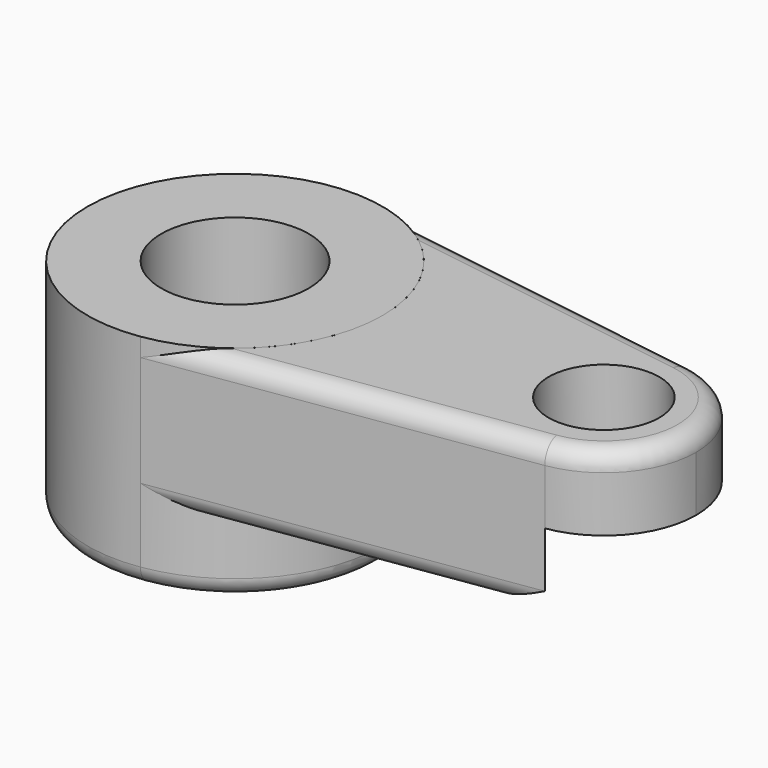
from build123d import *

# Parameters (mm, degrees)
F0_R         = 20
F1_DEPTH     = 60
F2_DEPTH     = 40
F0_R_2       = 15
F3_DEPTH     = 20
F4_R         = 5
F5_T1_DEPTH  = 141.3685996664
F5_T3_DEPTH  = 141.3685996664
F5_T5_DEPTH  = 120.1185996664
F5_T7_DEPTH  = 120.1185996664
F5_T10_ANGLE = 162.7461468826


# Not quite as in the source:
# - a fillet or chamfer that OpenCascade refuses, or shapes differently, is made with other operations: its cross-section is extruded or revolved along the edge and cut away or added
# - two fillets or chamfers of one size are made in one step


with BuildPart() as f1:
    # F0 (on Top) → F1 (new body)
    with BuildSketch(Plane.XY):
        with BuildLine():
            ThreePointArc((-44, -39.5474398666), (-19.6684982238, -26.0768096208), (-10, 0))
            ThreePointArc((-10, 0), (-19.6684982238, 26.0768096208), (-44, 39.5474398666))
            ThreePointArc((-44, 39.5474398666), (-90, 0), (-44, -39.5474398666))
        make_face()
        with Locations((-50, 0)):
            Circle(F0_R, mode=Mode.SUBTRACT)
    extrude(amount=-F1_DEPTH)

    # F4
    f4_edges = [f1.edges().sort_by_distance(p)[0] for p in [
        (-56, 39.54744, -60),
        (-70, 0, -60),
    ]]
    fillet(f4_edges, radius=F4_R)


with BuildPart() as f2:
    # F0 (on Top) → F2 (new body)
    with BuildSketch(Plane.XY):
        with BuildLine():
            ThreePointArc((-44, 39.5474398666), (-19.6684982238, 26.0768096208), (-10, 0))
            ThreePointArc((-10, 0), (-19.6684982238, -26.0768096208), (-44, -39.5474398666))
            Line((-44, -39.5474398666), (53.75, -24.7171499166))
            ThreePointArc((53.75, -24.7171499166), (25, 0), (53.75, 24.7171499166))
            Line((53.75, 24.7171499166), (-44, 39.5474398666))
        make_face()
    extrude(amount=-F2_DEPTH)

    # F0 (on Top) → F3 (join)
    with BuildSketch(Plane.XY):
        with BuildLine():
            ThreePointArc((75, 0), (68.9571886101, 16.298006013), (53.75, 24.7171499166))
            ThreePointArc((53.75, 24.7171499166), (25, 0), (53.75, -24.7171499166))
            ThreePointArc((53.75, -24.7171499166), (68.9571886101, -16.298006013), (75, 0))
        make_face()
        with Locations((50, 0)):
            Circle(F0_R_2, mode=Mode.SUBTRACT)
    extrude(amount=-F3_DEPTH)

    # F5: fillet of radius 5 on 9 edges, made by hand

    # F5_s2 → F5_t1 (cut)
    with BuildSketch(Plane(origin=(69.8845774291, -10.602644975, 0), x_dir=(0, 0, 1), z_dir=(-0.9886859967, 0.15, 0))):
        with BuildLine():
            ThreePointArc((-35, 32.5), (-38.5355339059, 31.0355339059), (-40, 27.5))
            Line((-40, 27.5), (-40, 32.5))
            Line((-40, 32.5), (-35, 32.5))
        make_face()
    extrude(amount=F5_T1_DEPTH, mode=Mode.SUBTRACT)

    # F5_s4 → F5_t3 (cut)
    with BuildSketch(Plane(origin=(-69.8845774291, -10.602644975, 0), x_dir=(0, 0, 1), z_dir=(0.9886859967, 0.15, 0))):
        with BuildLine():
            ThreePointArc((-40, 27.5), (-38.5355339059, 31.0355339059), (-35, 32.5))
            Line((-35, 32.5), (-40, 32.5))
            Line((-40, 32.5), (-40, 27.5))
        make_face()
    extrude(amount=F5_T3_DEPTH, mode=Mode.SUBTRACT)

    # F5_s6 → F5_t5 (cut)
    with BuildSketch(Plane(origin=(48.875, -7.415144975, 0), x_dir=(0, 0, 1), z_dir=(-0.9886859967, 0.15, 0))):
        with BuildLine():
            ThreePointArc((-5, 32.5), (-1.4644660941, 31.0355339059), (0, 27.5))
            Line((0, 27.5), (0, 32.5))
            Line((0, 32.5), (-5, 32.5))
        make_face()
    extrude(amount=F5_T5_DEPTH, mode=Mode.SUBTRACT)

    # F5_s8 → F5_t7 (cut)
    with BuildSketch(Plane(origin=(-69.8845774291, -10.602644975, 0), x_dir=(0, 0, 1), z_dir=(0.9886859967, 0.15, 0))):
        with BuildLine():
            ThreePointArc((-5, 32.5), (-1.4644660941, 31.0355339059), (0, 27.5))
            Line((0, 27.5), (0, 32.5))
            Line((0, 32.5), (-5, 32.5))
        make_face()
    extrude(amount=F5_T7_DEPTH, mode=Mode.SUBTRACT)

    # F5_s9 → F5_t10 (revolve, cut)
    with BuildSketch(Plane(origin=(48.875, -7.415144975, 0), x_dir=(0, 0, 1), z_dir=(-0.9886859967, 0.15, 0))):
        with BuildLine():
            ThreePointArc((-5, 32.5), (-1.4644660941, 31.0355339059), (0, 27.5))
            Line((0, 27.5), (0, 32.5))
            Line((0, 32.5), (-5, 32.5))
        make_face()
    revolve(axis=Axis((50, 0, 0), (0, 0, -1)), revolution_arc=F5_T10_ANGLE, mode=Mode.SUBTRACT)


solid = Compound([f1.part, f2.part])
